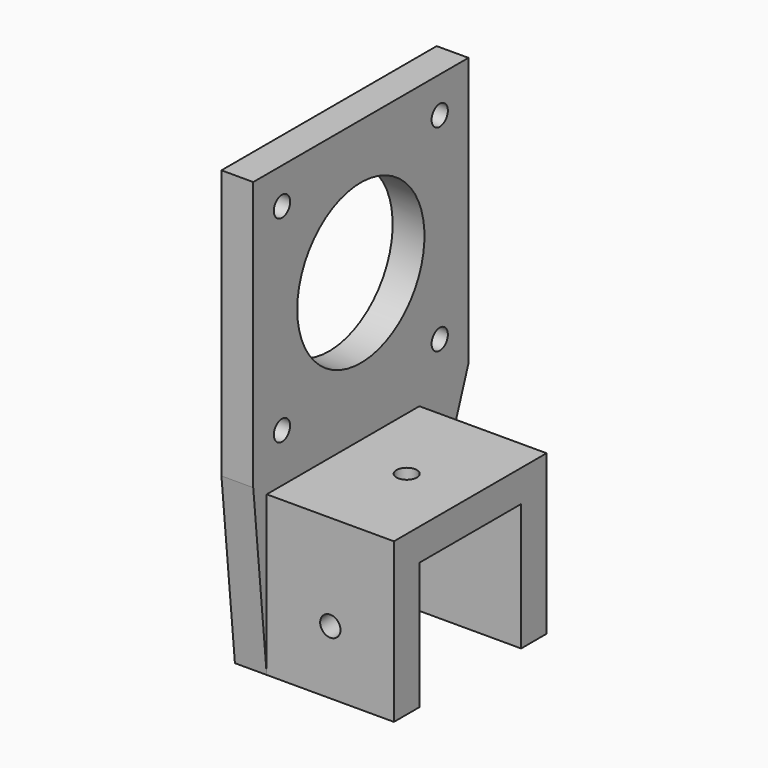
from build123d import *

# Parameters (mm, degrees)
F0_W       = 20
F0_H       = 25
F1_DEPTH   = 5
F2_W       = 20
F2_H       = 5
F3_DEPTH   = 20
F6_D       = 3.2
F6_ON_F5_D = 3.2
F7_W       = 20
F7_H       = 5
F8_DEPTH   = 25
F9_R       = 1.6
F9_R_2     = 12.5
F10_DEPTH  = 5


with BuildPart() as f1:
    # F0 (on Front) → F1 (new body)
    with BuildSketch(Plane.XZ):
        with Locations((10, 12.5)):
            Rectangle(F0_W, F0_H)
    extrude(amount=F1_DEPTH)

    # F2 (on face) → F3 (join)
    with BuildSketch(Plane(origin=(0, 0, 0), x_dir=(-1, 0, 0), z_dir=(0, 1, 0))):
        with Locations((-10, 22.5)):
            Rectangle(F2_W, F2_H)
    extrude(amount=F3_DEPTH)

    # F6 (through all)
    with Locations(Plane(origin=(0, 0, 0), x_dir=(-1, 0, 0), z_dir=(0, 1, 0))):
        with Locations((-10, 10)):
            Hole(F6_D / 2)

    # F6 on F5 (through all)
    with Locations(Plane(origin=(0, 0, 20), x_dir=(1, 0, 0), z_dir=(0, 0, -1))):
        with Locations((10, -10)):
            Hole(F6_ON_F5_D / 2)

    # F7 (on face) → F8 (join)
    with BuildSketch(Plane.XY.offset(25)):
        with Locations((10, 22.5)):
            Rectangle(F7_W, F7_H)
    extrude(amount=-F8_DEPTH)

    # F9 (on face) → F10 (join)
    with BuildSketch(Plane(origin=(0, 0, 0), x_dir=(0, -1, 0), z_dir=(-1, 0, 0))):
        Polygon((7.65, 27), (7.65, 69.3), (-34.65, 69.3), (-34.65, 27), (-25, 0), (-20, 0), (-20, 20), (0, 20), (0, 0), (5, 0), align=None)
        with Locations((-29, 32.65)):
            Circle(F9_R, mode=Mode.SUBTRACT)
        with Locations((2, 32.65)):
            Circle(F9_R, mode=Mode.SUBTRACT)
        with Locations((-29, 63.65)):
            Circle(F9_R, mode=Mode.SUBTRACT)
        with Locations((-13.5, 48.15)):
            Circle(F9_R_2, mode=Mode.SUBTRACT)
        with Locations((2, 63.65)):
            Circle(F9_R, mode=Mode.SUBTRACT)
    extrude(amount=F10_DEPTH)


solid = f1.part
